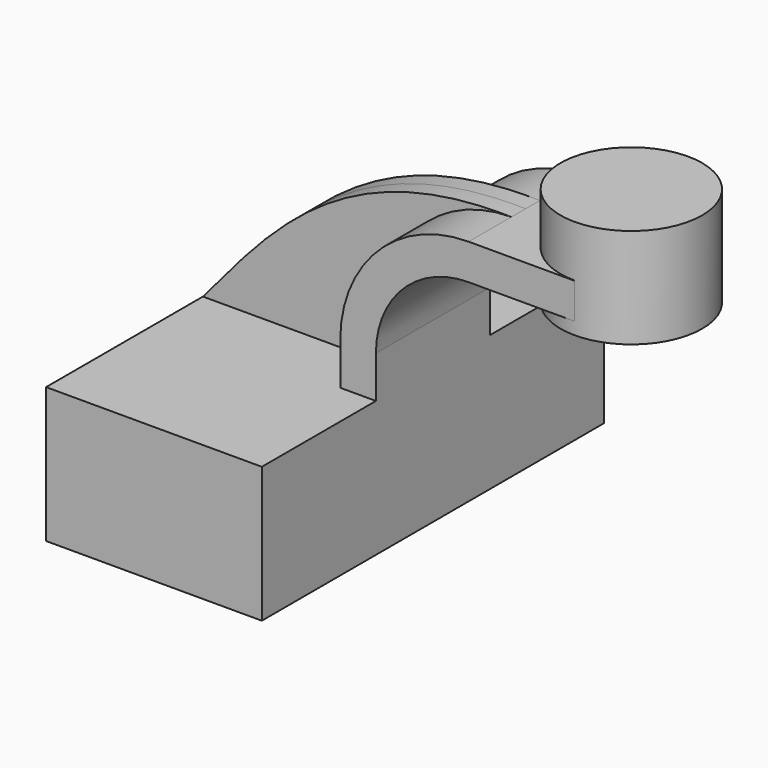
from build123d import *

# Parameters (mm, degrees)
F1_DEPTH = 76.2
F0_W     = 22.0843532517
F0_H     = 12.7000030306
F2_DEPTH = 25.4
F4_DEPTH = 6.35


# Not quite as in the source:
# - the program builds the solid bodies; features that only make, move or delete a surface that nothing else refers to are left out


with BuildPart() as f1:
    # F0 (on Front) → F1 (new body, symmetric)
    with BuildSketch(Plane.XZ):
        Polygon((30.5117662821, 21.1660526693), (-33.6534492671, 21.1660526693), (-33.6534492671, -27.1129291505), (43.2117693126, -27.1129291505), (43.2117693126, 21.1660526693), align=None)
    extrude(amount=F1_DEPTH, both=True)

    # F0 (on Front) → F2 (join, symmetric)
    with BuildSketch(Plane.XZ):
        with Locations((102.8505478717, 75.5138860928)):
            Rectangle(F0_W, F0_H)
        with BuildLine():
            Line((30.5117662821, 36.1293591958), (30.5117662821, 21.1660526693))
            Line((30.5117662821, 21.1660526693), (43.2117693126, 21.1660526693))
            Line((43.2117693126, 21.1660526693), (43.2117693126, 36.1293591958))
            ThreePointArc((43.2117693126, 36.1293591958), (52.8873577836, 59.4882961065), (76.2462946943, 69.1638845775))
            Line((76.2462946943, 69.1638845775), (91.8083712459, 69.1638845775))
            Line((91.8083712459, 69.1638845775), (91.8083712459, 81.8638876081))
            Line((91.8083712459, 81.8638876081), (76.2462946943, 81.8638876081))
            ThreePointArc((76.2462946943, 81.8638876081), (43.9070995196, 68.4685543705), (30.5117662821, 36.1293591958))
        make_face()
    extrude(amount=F2_DEPTH, both=True)

    # F0 (on Front) → F4 (join, symmetric)
    with BuildSketch(Plane.XZ):
        with BuildLine():
            add(Edge.make_bspline(
                [(-33.6534492671, 21.1660526693), (-9.9662784487, 49.1574853659), (15.5614716932, 83.2813158631), (76.2462946943, 81.8638876081)],
                knots=[0, 0, 0, 0, 125.5475244242, 125.5475244242, 125.5475244242, 125.5475244242], degree=3))
            Line((-33.6534492671, 21.1660526693), (30.5117662821, 21.1660526693))
            Line((30.5117662821, 21.1660526693), (30.5117662821, 36.1293591958))
            ThreePointArc((30.5117662821, 36.1293591958), (43.9070995196, 68.4685543705), (76.2462946943, 81.8638876081))
        make_face()
    extrude(amount=F4_DEPTH, both=True)

    # F0 (on Front) → F5 (revolve)
    with BuildSketch(Plane.XZ):
        Polygon((113.8927244975, 100.2546474338), (113.8927244975, 81.8638876081), (113.8927244975, 69.1638845775), (113.8927244975, 64.6806582808), (139.1344815493, 64.6806582808), (139.1344815493, 100.2546474338), align=None)
    revolve(axis=Axis((113.8927244975, 0, 84.7092660056), (0, 0, 1)))


solid = f1.part
